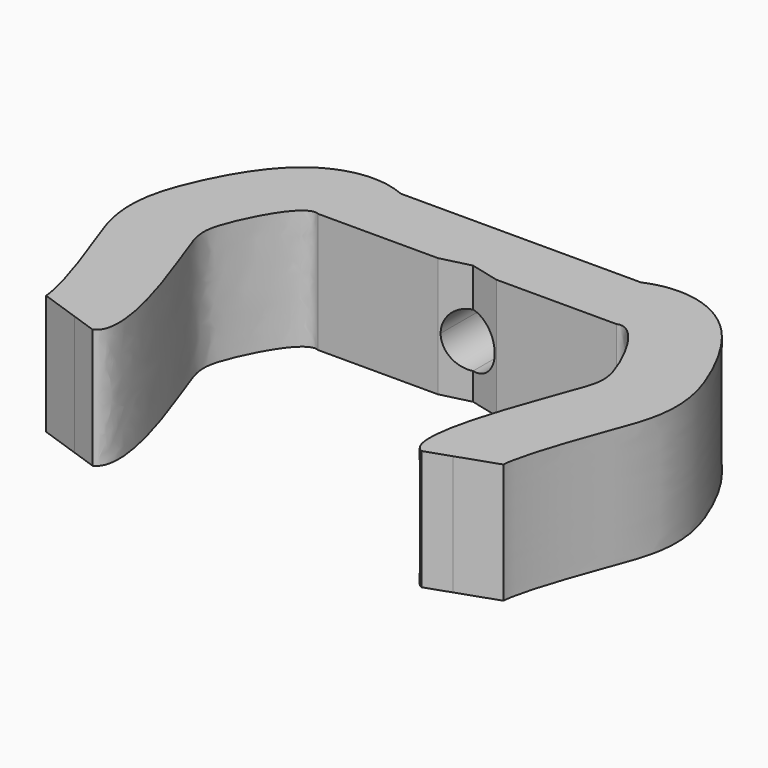
from build123d import *

# Parameters (mm, degrees)
F1_DEPTH = 8.2
F3_DEPTH = 25


# Not quite as in the source:
# - ends of sketch curves that miss each other by under 0.0002 mm in the source are joined
# - the dataset's text gives a spline's control points without its knots; the knots are read off the source's solid
# - a pattern or mirror of a feature is missing from the dataset's text; its kind, count and spacing are read off the source's solid


with BuildPart() as f1:
    # F0 (on Top) → F1 (new body)
    with BuildSketch(Plane.XY):
        with BuildLine():
            Line((-37.0359601621, 23.1417666937), (-35.029091494, 22.6463533197))
            Line((-35.029091494, 22.6463533197), (-26.829091494, 22.6463533197))
            add(Edge.make_bspline(
                [(-26.829091494, 22.6463533197), (-25.7721428325, 23.1219962444), (-22.9665433892, 17.8105744751), (-23.5981705487, 15.8048806569), (-27.5521563785, 5.4497575462), (-25.7911923863, 4.6763014154)],
                knots=[0, 0, 0, 0, 0.2521852928, 0.4666725674, 0.8252076015, 0.8252076015, 0.8252076015, 0.8252076015], degree=3))
            Line((-25.7911923863, 4.6763014154), (-24.099657673, 5.2599529941))
            Line((-24.099657673, 5.2599529941), (-21.4059092103, 6.1894110363))
            Line((-21.4059092103, 6.1894110363), (-21.4050641235, 6.1894110363))
            add(Edge.make_bspline(
                [(-28.8359559952, 27.225944927), (-28.4087434092, 27.4135047639), (-27.461802942, 27.6947287822), (-26.0417066535, 27.7257196671), (-24.8353649276, 27.4601249921), (-23.9004186629, 27.0585739987), (-23.1843370857, 26.6184702518), (-22.4373585387, 26.0340557803), (-21.7631698126, 25.3398551699), (-21.1480273409, 24.554901765), (-20.6408614836, 23.7924626862), (-20.2026828578, 23.0427855335), (-19.8169228918, 22.3051432259), (-19.476310452, 21.5835694031), (-19.2278267827, 21.0001643914), (-19.0488195155, 20.5420522561), (-18.8838554818, 20.0911409469), (-18.6895322517, 19.4935806167), (-18.4901693693, 18.6726095213), (-18.3664465965, 17.7432833331), (-18.3609909796, 16.7695348289), (-18.4708571085, 15.8577813838), (-18.6479909216, 15.0724194112), (-18.8479168659, 14.4060621583), (-19.0529170081, 13.8120761286), (-19.2281223024, 13.334340092), (-19.3753234655, 12.936696475), (-19.5305126309, 12.5179372236), (-19.7360371834, 11.9612723557), (-19.9942594284, 11.2495910041), (-20.2554944535, 10.5088037417), (-20.5108215915, 9.754945553), (-20.7509423149, 9.0060269452), (-20.9663871112, 8.282191306), (-21.1477182444, 7.6067669982), (-21.2628667399, 7.1076882355), (-21.3298297483, 6.7653175811), (-21.3670272177, 6.5431005017), (-21.3871822352, 6.3926980646), (-21.3973135938, 6.2977804421), (-21.4021997343, 6.2406673891), (-21.4042820534, 6.2069697584), (-21.4049161845, 6.1930561896), (-21.4050641235, 6.1894110363)],
                knots=[0.0003948374, 0.0003948374, 0.0003948374, 0.0003948374, 0.0116003267, 0.0232006534, 0.03480098, 0.0464013067, 0.0580016334, 0.0696019601, 0.0928026134, 0.1160032668, 0.1392039202, 0.1624045735, 0.1856052269, 0.2088058803, 0.2320065336, 0.2436068603, 0.255207187, 0.2784078403, 0.3016084937, 0.3248091471, 0.3480098004, 0.3712104538, 0.3944111071, 0.4176117605, 0.4408124139, 0.4640130672, 0.4756133939, 0.4872137206, 0.5104143739, 0.5336150273, 0.5568156807, 0.580016334, 0.6032169874, 0.6264176408, 0.6496182941, 0.6728189475, 0.6844192742, 0.6960196008, 0.7076199275, 0.7134200909, 0.7192202542, 0.7250204175, 0.7275315943, 0.7275315943, 0.7275315943, 0.7275315943], degree=3))
            Line((-28.8359559952, 27.225944927), (-37.0359601621, 27.2259544187))
            Line((-37.0359601621, 27.2259544187), (-37.0359601621, 23.1417666937))
        make_face()
    extrude(amount=F1_DEPTH)

    # F1_copies: F1 across plane


with BuildPart() as f1_1:
    add(f1.part)
    add(f1.part.mirror(Plane(origin=(-37.03596, 0, 0), x_dir=(0, 0, -1), z_dir=(-1, 0, 0))))

    # F2 (on face) → F3 (cut)
    with BuildSketch(Plane(origin=(0, 27.2259544187, 0), x_dir=(-1, 0, 0), z_dir=(0, 1, 0))):
        with BuildLine():
            Line((37.0359601621, 1.852566959), (37.0359601621, 5.552566959))
            ThreePointArc((37.0359601621, 5.552566959), (35.1859601621, 3.702566959), (37.0359601621, 1.852566959))
        make_face()
        with BuildLine():
            ThreePointArc((37.0359601621, 1.852566959), (38.3441077073, 2.3944194138), (38.8859601621, 3.702566959))
            ThreePointArc((38.8859601621, 3.702566959), (38.3441077073, 5.0107145042), (37.0359601621, 5.552566959))
            Line((37.0359601621, 5.552566959), (37.0359601621, 1.852566959))
        make_face()
    extrude(amount=-F3_DEPTH, mode=Mode.SUBTRACT)


solid = f1_1.part
